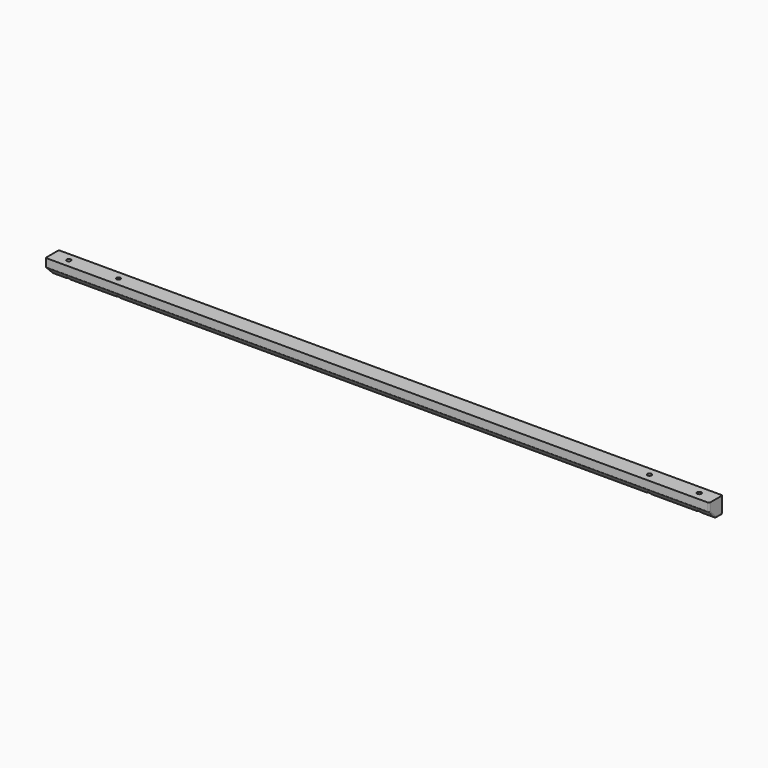
from build123d import *

# Parameters (mm, degrees)
F0_W         = 508
F0_H         = 12.7
F0_R         = 1.5875
F1_DEPTH     = 6.35
F2_T1_DEPTH  = 540.6603739472
F3_T1_DEPTH  = 8.3226920908
F3_T3_DEPTH  = 8.0055929849
F3_T5_DEPTH  = 5.2274679849
F3_T7_DEPTH  = 13.890625
F3_T9_DEPTH  = 8.3226920908
F3_T11_DEPTH = 506.4125
F3_T13_DEPTH = 11.1407050378
F3_T15_DEPTH = 36.5689100757
F3_T17_DEPTH = 11.1407050378
F3_T22_DEPTH = 0.809625
F3_T28_DEPTH = 0.809625
F3_S33_W     = 0.809625
F3_S33_H     = 0.809625
F3_T34_DEPTH = 0.809625
F3_T40_DEPTH = 0.809625
F3_T46_DEPTH = 0.809625
F3_S51_W     = 0.809625
F3_S51_H     = 0.809625
F3_T52_DEPTH = 0.809625


# Not quite as in the source:
# - a fillet or chamfer that OpenCascade refuses, or shapes differently, is made with other operations: its cross-section is extruded or revolved along the edge and cut away or added


with BuildPart() as f1:
    # F0 (on Top) → F1 (new body, symmetric)
    with BuildSketch(Plane.XY):
        with Locations((4.392349353, 0)):
            Rectangle(F0_W, F0_H)
        with Locations((-236.907650647, 0)):
            Circle(F0_R, mode=Mode.SUBTRACT)
        with Locations((-198.807650647, 0)):
            Circle(F0_R, mode=Mode.SUBTRACT)
        with Locations((207.592349353, 0)):
            Circle(F0_R, mode=Mode.SUBTRACT)
        with Locations((245.692349353, 0)):
            Circle(F0_R, mode=Mode.SUBTRACT)
    extrude(amount=F1_DEPTH, both=True)

    # F2: chamfer of 6.35 on 1 edges, made by hand

    # F2_s2 → F2_t1 (cut)
    with BuildSketch(Plane.YZ.offset(-265.9378376206)):
        Polygon((-6.35, 0), (0, -6.35), (-6.35, -6.35), align=None)
    extrude(amount=F2_T1_DEPTH, mode=Mode.SUBTRACT)

    # F3: fillet of radius 0.79375 on 13 edges, made by hand

    # F3_s2 → F3_t1 (cut)
    with BuildSketch(Plane(origin=(0, 2.9425160076, -2.9425160076), x_dir=(1, 0, 0), z_dir=(0, -0.7071067812, 0.7071067812))):
        with BuildLine():
            ThreePointArc((258.392349353, -3.6963780605), (258.1598653606, -4.2576440681), (257.598599353, -4.4901280605))
            Line((257.598599353, -4.4901280605), (258.392349353, -4.4901280605))
            Line((258.392349353, -4.4901280605), (258.392349353, -3.6963780605))
        make_face()
    extrude(amount=F3_T1_DEPTH, mode=Mode.SUBTRACT)

    # F3_s4 → F3_t3 (cut)
    with BuildSketch(Plane.XY.offset(0.3287820151)):
        with BuildLine():
            ThreePointArc((258.392349353, -5.55625), (258.1598653606, -6.1175160076), (257.598599353, -6.35))
            Line((257.598599353, -6.35), (258.392349353, -6.35))
            Line((258.392349353, -6.35), (258.392349353, -5.55625))
        make_face()
        with BuildLine():
            ThreePointArc((-249.607650647, -5.55625), (-249.3751666546, -6.1175160076), (-248.813900647, -6.35))
            Line((-248.813900647, -6.35), (-249.607650647, -6.35))
            Line((-249.607650647, -6.35), (-249.607650647, -5.55625))
        make_face()
    extrude(amount=F3_T3_DEPTH, mode=Mode.SUBTRACT)

    # F3_s6 → F3_t5 (cut)
    with BuildSketch(Plane.XZ.offset(-5.55625)):
        with BuildLine():
            ThreePointArc((257.598599353, -6.35), (258.1598653606, -6.1175160076), (258.392349353, -5.55625))
            Line((258.392349353, -5.55625), (258.392349353, -6.35))
            Line((258.392349353, -6.35), (257.598599353, -6.35))
        make_face()
        with BuildLine():
            ThreePointArc((-248.813900647, -6.35), (-249.3751666546, -6.1175160076), (-249.607650647, -5.55625))
            Line((-249.607650647, -5.55625), (-249.607650647, -6.35))
            Line((-249.607650647, -6.35), (-248.813900647, -6.35))
        make_face()
    extrude(amount=F3_T5_DEPTH, mode=Mode.SUBTRACT)

    # F3_s8 → F3_t7 (cut)
    with BuildSketch(Plane.XY.offset(-5.55625)):
        with BuildLine():
            ThreePointArc((257.598599353, 6.35), (258.1598653606, 6.1175160076), (258.392349353, 5.55625))
            Line((258.392349353, 5.55625), (258.392349353, 6.35))
            Line((258.392349353, 6.35), (257.598599353, 6.35))
        make_face()
        with BuildLine():
            ThreePointArc((-248.813900647, 6.35), (-249.3751666546, 6.1175160076), (-249.607650647, 5.55625))
            Line((-249.607650647, 5.55625), (-249.607650647, 6.35))
            Line((-249.607650647, 6.35), (-248.813900647, 6.35))
        make_face()
    extrude(amount=F3_T7_DEPTH, mode=Mode.SUBTRACT)

    # F3_s10 → F3_t9 (cut)
    with BuildSketch(Plane(origin=(0, -2.9425160076, 2.9425160076), x_dir=(1, 0, 0), z_dir=(0, 0.7071067812, -0.7071067812))):
        with BuildLine():
            ThreePointArc((-249.607650647, 3.6963780605), (-249.3751666546, 4.2576440681), (-248.813900647, 4.4901280605))
            Line((-248.813900647, 4.4901280605), (-249.607650647, 4.4901280605))
            Line((-249.607650647, 4.4901280605), (-249.607650647, 3.6963780605))
        make_face()
    extrude(amount=F3_T9_DEPTH, mode=Mode.SUBTRACT)

    # F3_s12 → F3_t11 (cut)
    with BuildSketch(Plane.YZ.offset(-248.813900647)):
        with BuildLine():
            ThreePointArc((-6.1175160076, -0.2324839924), (-6.2895793789, 0.0250270407), (-6.35, 0.3287820151))
            Line((-6.35, 0.3287820151), (-6.35, 0))
            Line((-6.35, 0), (-6.1175160076, -0.2324839924))
        make_face()
        with BuildLine():
            ThreePointArc((6.35, -5.55625), (6.1175160076, -6.1175160076), (5.55625, -6.35))
            Line((5.55625, -6.35), (6.35, -6.35))
            Line((6.35, -6.35), (6.35, -5.55625))
        make_face()
    extrude(amount=F3_T11_DEPTH, mode=Mode.SUBTRACT)

    # F3_s14 → F3_t13 (cut)
    with BuildSketch(Plane.YZ.offset(-248.813900647)):
        with BuildLine():
            ThreePointArc((0.3287820151, -6.35), (0.0250270407, -6.2895793789), (-0.2324839924, -6.1175160076))
            Line((-0.2324839924, -6.1175160076), (0, -6.35))
            Line((0, -6.35), (0.3287820151, -6.35))
        make_face()
    extrude(amount=F3_T13_DEPTH, mode=Mode.SUBTRACT)

    # F3_s16 → F3_t15 (cut)
    with BuildSketch(Plane.YZ.offset(-236.1421056848)):
        with BuildLine():
            ThreePointArc((0.3287820151, -6.35), (0.0250270407, -6.2895793789), (-0.2324839924, -6.1175160076))
            Line((-0.2324839924, -6.1175160076), (0, -6.35))
            Line((0, -6.35), (0.3287820151, -6.35))
        make_face()
    extrude(amount=F3_T15_DEPTH, mode=Mode.SUBTRACT)

    # F3_s18 → F3_t17 (cut)
    with BuildSketch(Plane.YZ.offset(246.4578943152)):
        with BuildLine():
            ThreePointArc((0.3287820151, -6.35), (0.0250270407, -6.2895793789), (-0.2324839924, -6.1175160076))
            Line((-0.2324839924, -6.1175160076), (0, -6.35))
            Line((0, -6.35), (0.3287820151, -6.35))
        make_face()
    extrude(amount=F3_T17_DEPTH, mode=Mode.SUBTRACT)


with BuildPart() as f3_tool20:
    # F3_s21 → F3_t22 (new body)
    with BuildSketch(Plane.YZ.offset(257.598599353)):
        Polygon((0.3287820151, -5.55625), (-0.2437093126, -6.1287413277), (-0.0065756403, -6.365875), (0.3287820151, -6.365875), align=None)
    extrude(amount=F3_T22_DEPTH)

    # F3_s23 → F3_t24 (revolve, cut)
    with BuildSketch(Plane(origin=(257.598599353, 0.3287820151, -5.55625), x_dir=(0, 0.3826834324, 0.9238795325), z_dir=(0, 0.9238795325, -0.3826834324))):
        with BuildLine():
            ThreePointArc((0, -0.79375), (0.79375, 0), (0, 0.79375))
            Line((0, 0.79375), (0, -0.79375))
        make_face()
    revolve(axis=Axis((257.598599353, 0.3287820151, -5.55625), (1, 0, 0)), mode=Mode.SUBTRACT)


with BuildPart() as f1_1:
    add(f1.part)

    # F3_t19: cut F3_tool20
    add(f3_tool20.part, mode=Mode.SUBTRACT)


with BuildPart() as f3_tool26:
    # F3_s27 → F3_t28 (new body)
    with BuildSketch(Plane.YZ.offset(257.598599353)):
        Polygon((-5.55625, 0.3287820151), (-6.1287413277, -0.2437093126), (-6.365875, -0.0065756403), (-6.365875, 0.3287820151), align=None)
    extrude(amount=F3_T28_DEPTH)

    # F3_s29 → F3_t30 (revolve, cut)
    with BuildSketch(Plane(origin=(257.598599353, -5.55625, 0.3287820151), x_dir=(0, 0.9238795325, 0.3826834324), z_dir=(0, 0.3826834324, -0.9238795325))):
        with BuildLine():
            ThreePointArc((0, -0.79375), (0.79375, 0), (0, 0.79375))
            Line((0, 0.79375), (0, -0.79375))
        make_face()
    revolve(axis=Axis((257.598599353, -5.55625, 0.3287820151), (1, 0, 0)), mode=Mode.SUBTRACT)


with BuildPart() as f1_2:
    add(f1_1.part)

    # F3_t25: cut F3_tool26
    add(f3_tool26.part, mode=Mode.SUBTRACT)


with BuildPart() as f3_tool32:
    # F3_s33 → F3_t34 (new body)
    with BuildSketch(Plane.XZ.offset(-5.55625)):
        with Locations((258.003411853, -5.9610625)):
            Rectangle(F3_S33_W, F3_S33_H)
    extrude(amount=-F3_T34_DEPTH)

    # F3_s35 → F3_t36 (revolve, cut)
    with BuildSketch(Plane(origin=(257.598599353, 5.55625, -5.55625), x_dir=(-0.7071067812, 0, 0.7071067812), z_dir=(-0.7071067812, 0, -0.7071067812))):
        with BuildLine():
            ThreePointArc((0, -0.79375), (0.79375, 0), (0, 0.79375))
            Line((0, 0.79375), (0, -0.79375))
        make_face()
    revolve(axis=Axis((257.598599353, 5.55625, -5.55625), (0, 1, 0)), mode=Mode.SUBTRACT)


with BuildPart() as f1_3:
    add(f1_2.part)

    # F3_t31: cut F3_tool32
    add(f3_tool32.part, mode=Mode.SUBTRACT)


with BuildPart() as f3_tool38:
    # F3_s39 → F3_t40 (new body)
    with BuildSketch(Plane.YZ.offset(-248.813900647)):
        Polygon((-5.55625, 0.3287820151), (-6.365875, 0.3287820151), (-6.365875, -0.0065756403), (-6.1287413277, -0.2437093126), align=None)
    extrude(amount=-F3_T40_DEPTH)

    # F3_s41 → F3_t42 (revolve, cut)
    with BuildSketch(Plane(origin=(-248.813900647, -5.55625, 0.3287820151), x_dir=(0, 0.9238795325, 0.3826834324), z_dir=(0, -0.3826834324, 0.9238795325))):
        with BuildLine():
            ThreePointArc((0, -0.79375), (0.79375, 0), (0, 0.79375))
            Line((0, 0.79375), (0, -0.79375))
        make_face()
    revolve(axis=Axis((-248.813900647, -5.55625, 0.3287820151), (-1, 0, 0)), mode=Mode.SUBTRACT)


with BuildPart() as f1_4:
    add(f1_3.part)

    # F3_t37: cut F3_tool38
    add(f3_tool38.part, mode=Mode.SUBTRACT)


with BuildPart() as f3_tool44:
    # F3_s45 → F3_t46 (new body)
    with BuildSketch(Plane.YZ.offset(-248.813900647)):
        Polygon((0.3287820151, -5.55625), (-0.2437093126, -6.1287413277), (-0.0065756403, -6.365875), (0.3287820151, -6.365875), align=None)
    extrude(amount=-F3_T46_DEPTH)

    # F3_s47 → F3_t48 (revolve, cut)
    with BuildSketch(Plane(origin=(-248.813900647, 0.3287820151, -5.55625), x_dir=(0, 0.3826834324, 0.9238795325), z_dir=(0, -0.9238795325, 0.3826834324))):
        with BuildLine():
            ThreePointArc((0, -0.79375), (0.79375, 0), (0, 0.79375))
            Line((0, 0.79375), (0, -0.79375))
        make_face()
    revolve(axis=Axis((-248.813900647, 0.3287820151, -5.55625), (-1, 0, 0)), mode=Mode.SUBTRACT)


with BuildPart() as f1_5:
    add(f1_4.part)

    # F3_t43: cut F3_tool44
    add(f3_tool44.part, mode=Mode.SUBTRACT)


with BuildPart() as f3_tool50:
    # F3_s51 → F3_t52 (new body)
    with BuildSketch(Plane.XZ.offset(-5.55625)):
        with Locations((-249.218713147, -5.9610625)):
            Rectangle(F3_S51_W, F3_S51_H)
    extrude(amount=-F3_T52_DEPTH)

    # F3_s53 → F3_t54 (revolve, cut)
    with BuildSketch(Plane(origin=(-248.813900647, 5.55625, -5.55625), x_dir=(0.7071067812, 0, 0.7071067812), z_dir=(-0.7071067812, 0, 0.7071067812))):
        with BuildLine():
            ThreePointArc((0, -0.79375), (0.79375, 0), (0, 0.79375))
            Line((0, 0.79375), (0, -0.79375))
        make_face()
    revolve(axis=Axis((-248.813900647, 5.55625, -5.55625), (0, 1, 0)), mode=Mode.SUBTRACT)


with BuildPart() as f1_6:
    add(f1_5.part)

    # F3_t49: cut F3_tool50
    add(f3_tool50.part, mode=Mode.SUBTRACT)


solid = f1_6.part
